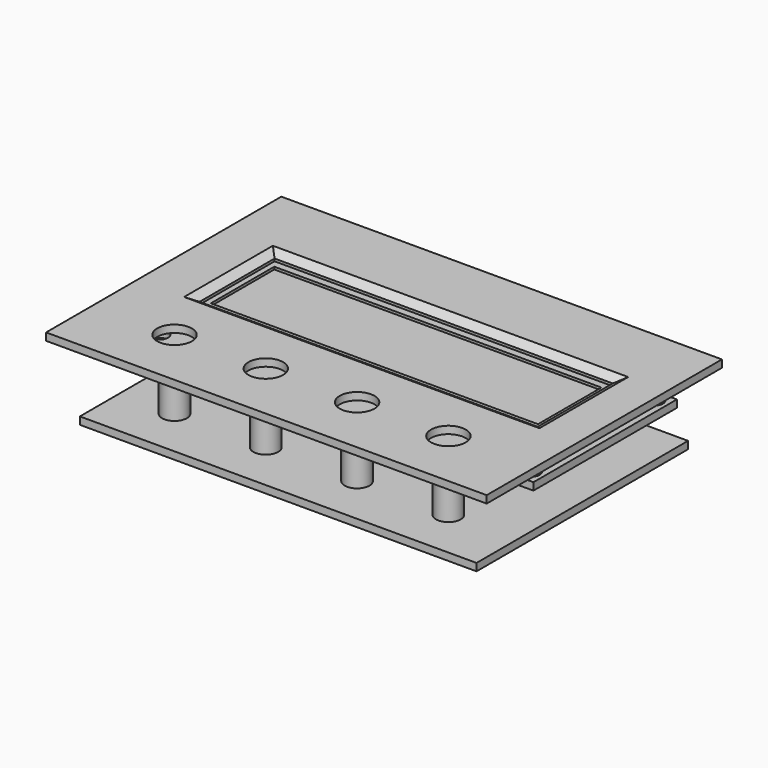
from build123d import *

# Parameters (mm, degrees)
F0_W      = 80.01
F0_H      = 36.068
F0_W_2    = 71.247
F0_H_2    = 25.019
F0_W_3    = 66.04
F0_H_3    = 16.002
F0_H_4    = 14.351
F0_R      = 2.5
F0_H_5    = 2.921
F1_DEPTH  = 1.5
F2_DEPTH  = 10
F4_W      = 80.01
F4_H      = 36.1823
F4_R      = 1.75
F5_DEPTH  = 1.5
F6_W      = 71.12
F6_H      = 25.146
F6_W_2    = 66
F6_H_2    = 16
F7_DEPTH  = 4
F8_DEPTH  = 3.5
F9_W      = 88.8787768781
F9_H      = 59.3131650239
F9_R      = 3.5
F9_W_2    = 71.12
F9_H_2    = 25.146
F9_W_3    = 68.2152619944
F9_H_3    = 18.9172932116
F10_DEPTH = 1.5
F11_SIZE2 = 1.7320508076
F11_SIZE  = 1


# Not quite as in the source:
# - a feature of the source that left no trace in its solid (it failed there, or was rolled back) is left out


with BuildPart() as f1:
    # F0 (on Top) → F1 (new body)
    with BuildSketch(Plane.XY):
        with Locations((-17.3261313879, 1.0963964765)):
            Rectangle(F0_W, F0_H)
        with Locations((-17.2626313879, 1.0328964765)):
            Rectangle(F0_W_2, F0_H_2, mode=Mode.SUBTRACT)
        with Locations((-17.2626313879, 1.0328964765)):
            Rectangle(F0_W_2, F0_H_2)
        with Locations((-17.1991313879, 1.0963964765)):
            Rectangle(F0_W_3, F0_H_3, mode=Mode.SUBTRACT)
        with Locations((-17.3261313879, -24.1131035235)):
            Rectangle(F0_W, F0_H_4)
        with Locations((-46.2821313879, -21.2417540622)):
            Circle(F0_R, mode=Mode.SUBTRACT)
        with Locations((-27.8671313879, -21.2417540622)):
            Circle(F0_R, mode=Mode.SUBTRACT)
        with Locations((-9.4521313879, -21.2417540622)):
            Circle(F0_R, mode=Mode.SUBTRACT)
        with Locations((8.9628686121, -21.2417540622)):
            Circle(F0_R, mode=Mode.SUBTRACT)
        with Locations((-17.1991313879, 1.0963964765)):
            Rectangle(F0_W_3, F0_H_3)
        with Locations((-17.3261313879, 20.5908964765)):
            Rectangle(F0_W, F0_H_5)
        with Locations((-9.4521313879, -21.2417540622)):
            Circle(F0_R)
        with Locations((-46.2821313879, -21.2417540622)):
            Circle(F0_R)
        with Locations((-27.8671313879, -21.2417540622)):
            Circle(F0_R)
        with Locations((8.9628686121, -21.2417540622)):
            Circle(F0_R)
    extrude(amount=-F1_DEPTH)


with BuildPart() as f2:
    # F0 (on Top) → F2 (new body)
    with BuildSketch(Plane.XY):
        with Locations((-46.2821313879, -21.2417540622)):
            Circle(F0_R)
    extrude(amount=F2_DEPTH)


with BuildPart() as f2b:
    # F0 (on Top) → F2, piece 2 (new body)
    with BuildSketch(Plane.XY):
        with Locations((-27.8671313879, -21.2417540622)):
            Circle(F0_R)
    extrude(amount=F2_DEPTH)


with BuildPart() as f2c:
    # F0 (on Top) → F2, piece 3 (new body)
    with BuildSketch(Plane.XY):
        with Locations((-9.4521313879, -21.2417540622)):
            Circle(F0_R)
    extrude(amount=F2_DEPTH)


with BuildPart() as f2d:
    # F0 (on Top) → F2, piece 4 (new body)
    with BuildSketch(Plane.XY):
        with Locations((8.9628686121, -21.2417540622)):
            Circle(F0_R)
    extrude(amount=F2_DEPTH)


with BuildPart() as f5:
    # F4 (on offset) → F5 (new body)
    with BuildSketch(Plane.XY.offset(7)):
        with Locations((-17.3261313879, 1.1535464765)):
            Rectangle(F4_W, F4_H)
        with Locations((-54.7911313879, -14.3976035235)):
            Circle(F4_R, mode=Mode.SUBTRACT)
        with Locations((20.1388686121, -14.3976035235)):
            Circle(F4_R, mode=Mode.SUBTRACT)
        with Locations((-54.7911313879, 16.7046964765)):
            Circle(F4_R, mode=Mode.SUBTRACT)
        with Locations((20.1388686121, 16.7046964765)):
            Circle(F4_R, mode=Mode.SUBTRACT)
    extrude(amount=F5_DEPTH)


with BuildPart() as f7:
    # F6 (on face) → F7 (new body)
    with BuildSketch(Plane.XY.offset(8.5)):
        with Locations((-17.3261313879, 0.9693964765)):
            Rectangle(F6_W, F6_H)
        with Locations((-17.3261313879, 0.9693964765)):
            Rectangle(F6_W_2, F6_H_2, mode=Mode.SUBTRACT)
    extrude(amount=F7_DEPTH)


with BuildPart() as f8:
    # F6 (on face) → F8 (new body)
    with BuildSketch(Plane.XY.offset(8.5)):
        with Locations((-17.3261313879, 0.9693964765)):
            Rectangle(F6_W_2, F6_H_2)
    extrude(amount=F8_DEPTH)


with BuildPart() as f10:
    # F9 (on face) → F10 (new body)
    with BuildSketch(Plane.XY.offset(12.5)):
        with Locations((-18.1514117867, -3.5815080628)):
            Rectangle(F9_W, F9_H)
        with Locations((-46.2821313879, -21.2417540622)):
            Circle(F9_R, mode=Mode.SUBTRACT)
        with Locations((-27.8671313879, -21.2417540622)):
            Circle(F9_R, mode=Mode.SUBTRACT)
        with Locations((-9.4521313879, -21.2417540622)):
            Circle(F9_R, mode=Mode.SUBTRACT)
        with Locations((8.9628686121, -21.2417540622)):
            Circle(F9_R, mode=Mode.SUBTRACT)
        with Locations((-17.3261313879, 0.9693964765)):
            Rectangle(F9_W_2, F9_H_2, mode=Mode.SUBTRACT)
        with Locations((-17.3261313879, 0.9693964765)):
            Rectangle(F9_W_2, F9_H_2)
        with Locations((-17.3261313879, 0.9693964765)):
            Rectangle(F9_W_3, F9_H_3, mode=Mode.SUBTRACT)
    extrude(amount=F10_DEPTH)

    # F11
    f11_edges = [f10.edges().sort_by_distance(p)[0] for p in [
        (-17.326131, 10.428043, 14),
        (-51.433762, 0.969396, 14),
        (-17.326131, -8.48925, 14),
        (16.7815, 0.969396, 14),
    ]]
    chamfer(f11_edges, length=F11_SIZE, length2=F11_SIZE2)


solid = Compound([f1.part, f2.part, f2b.part, f2c.part, f2d.part, f5.part, f7.part, f8.part, f10.part])
